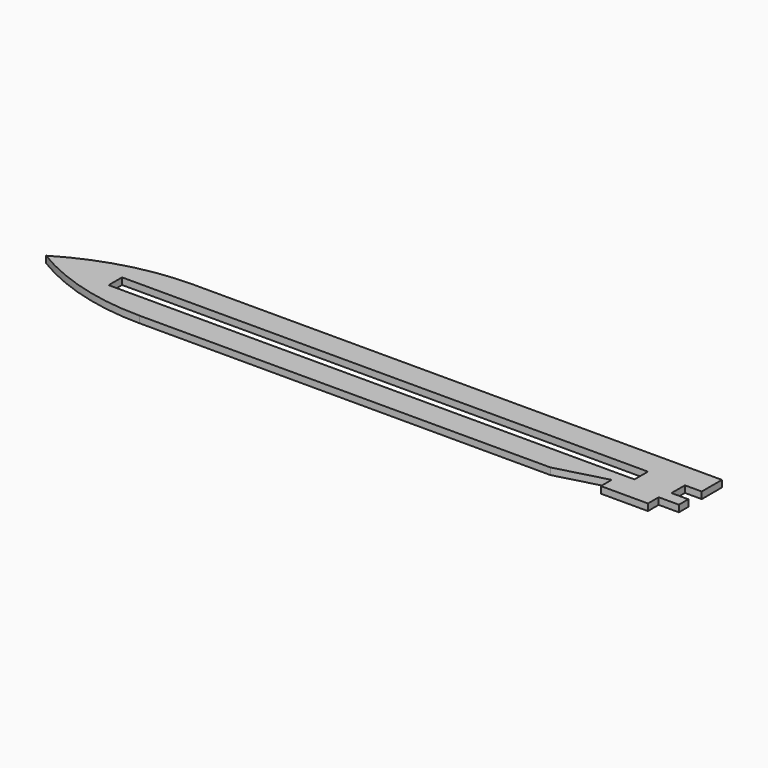
from build123d import *

# Parameters (mm, degrees)
F0_W        = 193
F0_H        = 20
F1_DEPTH    = 2
F2_W        = 5
F2_H        = 5
F2_W_2      = 167
F3_DEPTH    = 25
F4_SIZE2    = 14.99999
F4_SIZE     = 9.99999
F5_W        = 6
F5_H        = 4
F6_DEPTH    = 25
F7_T1_DEPTH = 106.0916256943
F8_DEPTH    = 10.6


# Not quite as in the source:
# - a fillet or chamfer that OpenCascade refuses, or shapes differently, is made with other operations: its cross-section is extruded or revolved along the edge and cut away or added
# - a fillet or chamfer is up to 0.001 mm smaller than in the source, because OpenCascade refuses the exact size


with BuildPart() as f1:
    # F0 (on Top) → F1 (new body)
    with BuildSketch(Plane.XY):
        Rectangle(F0_W, F0_H)
    extrude(amount=F1_DEPTH)

    # F2 (on face) → F3 (cut)
    with BuildSketch(Plane.XY.offset(2)):
        with Locations((94, 0)):
            Rectangle(F2_W, F2_H)
        with Locations((-3, 0)):
            Rectangle(F2_W_2, F2_H)
    extrude(amount=-F3_DEPTH, mode=Mode.SUBTRACT)

    # F4 (size 10 and 15 in the source; OpenCascade refuses exactly that, so slightly less here)
    f4_edges = [f1.edges().sort_by_distance(p)[0] for p in [
        (-96.5, 10, 1),
        (-96.5, -10, 1),
    ]]
    f4_side = f1.faces().sort_by_distance((-96.5, 0, 1))[0]
    chamfer(f4_edges, length=F4_SIZE, length2=F4_SIZE2, reference=f4_side)

    # F5 (on face) → F6 (cut)
    with BuildSketch(Plane.XY.offset(2)):
        with Locations((93.5, -8)):
            Rectangle(F5_W, F5_H)
        Polygon((61.5, -10), (76.5, -10), (76.5, -6), align=None)
    extrude(amount=-F6_DEPTH, mode=Mode.SUBTRACT)

    # F7: fillet of radius 69.147644117 on 2 edges, made by hand

    # F7_s2 → F7_t1 (cut)
    with BuildSketch(Plane.XY.offset(-52.0458128472)):
        with BuildLine():
            ThreePointArc((-96.5, -1e-05), (-79.2757127961, -7.4530977113), (-60.6816848611, -10))
            Line((-60.6816848611, -10), (-81.50001, -10))
            Line((-81.50001, -10), (-96.5, -1e-05))
        make_face()
        with BuildLine():
            ThreePointArc((-96.5, 1e-05), (-79.2757127961, 7.4530977113), (-60.6816848611, 10))
            Line((-60.6816848611, 10), (-81.50001, 10))
            Line((-81.50001, 10), (-96.5, 1e-05))
        make_face()
    extrude(amount=F7_T1_DEPTH, mode=Mode.SUBTRACT)

    # F8 (add): a face of the model
    f8_faces = [f1.faces().sort_by_distance(p)[0] for p in [
        (-86.5, 0, 1),
    ]]
    extrude(f8_faces, amount=F8_DEPTH)


solid = f1.part
